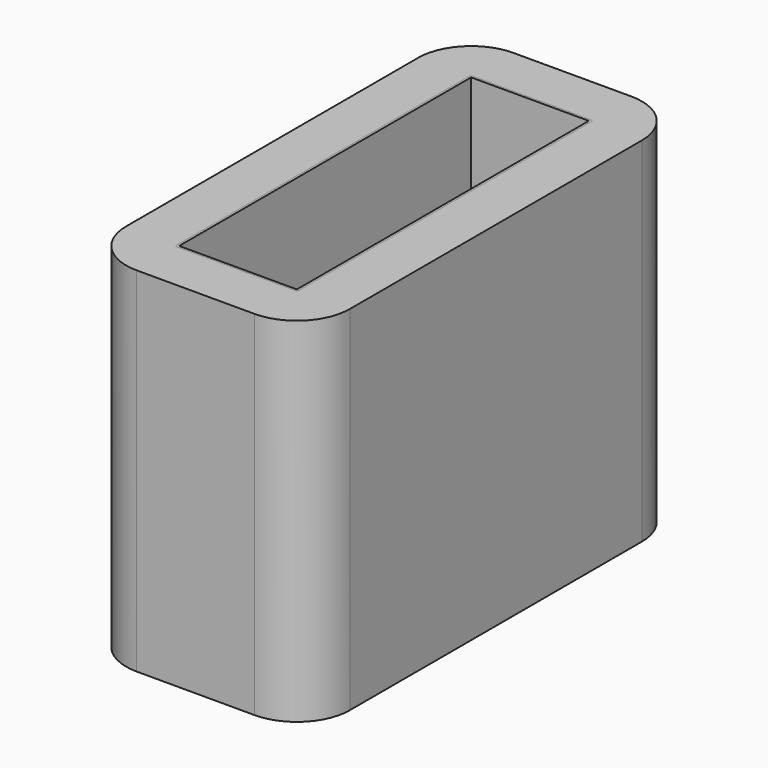
from build123d import *

# Parameters (mm, degrees)
F4_W      = 72.39
F4_H      = 152.4
F5_DEPTH  = 114.3
F6_R      = 17.145
F7_W      = 39.624
F7_H      = 119.634
F8_DEPTH  = 114.3
F9_W      = 39.624
F9_H      = 119.634
F10_DEPTH = 114.3
F11_W     = 38.1
F11_H     = 118.11
F12_DEPTH = 114.3
F13_R     = 0.762
F14_R     = 0.762


with BuildPart() as f5:
    # F4 (on Top) → F5 (new body)
    with BuildSketch(Plane.XY):
        Rectangle(F4_W, F4_H)
    extrude(amount=-F5_DEPTH)

    # F6
    f6_edges = [f5.edges().sort_by_distance(p)[0] for p in [
        (-36.195, 76.2, -57.15),
        (36.195, 76.2, -57.15),
        (36.195, -76.2, -57.15),
        (-36.195, -76.2, -57.15),
    ]]
    fillet(f6_edges, radius=F6_R)

    # F7 (on face) → F8 (cut)
    with BuildSketch(Plane.XY):
        Rectangle(F7_W, F7_H)
    extrude(amount=-F8_DEPTH, mode=Mode.SUBTRACT)

    # F14
    f14_edges = [f5.edges().sort_by_distance(p)[0] for p in [
        (-19.812, 59.817, -57.15),
        (-19.812, -59.817, -57.15),
        (19.812, -59.817, -57.15),
        (19.812, 59.817, -57.15),
    ]]
    fillet(f14_edges, radius=F14_R)


with BuildPart() as f10:
    # F9 (on face) → F10 (new body)
    with BuildSketch(Plane.XY):
        Rectangle(F9_W, F9_H)
    extrude(amount=-F10_DEPTH)

    # F11 (on face) → F12 (cut)
    with BuildSketch(Plane.XY):
        Rectangle(F11_W, F11_H)
    extrude(amount=-F12_DEPTH, mode=Mode.SUBTRACT)

    # F13
    f13_edges = [f10.edges().sort_by_distance(p)[0] for p in [
        (-19.812, 59.817, -57.15),
        (19.812, 59.817, -57.15),
        (19.812, -59.817, -57.15),
        (-19.812, -59.817, -57.15),
    ]]
    fillet(f13_edges, radius=F13_R)


solid = Compound([f5.part, f10.part])
